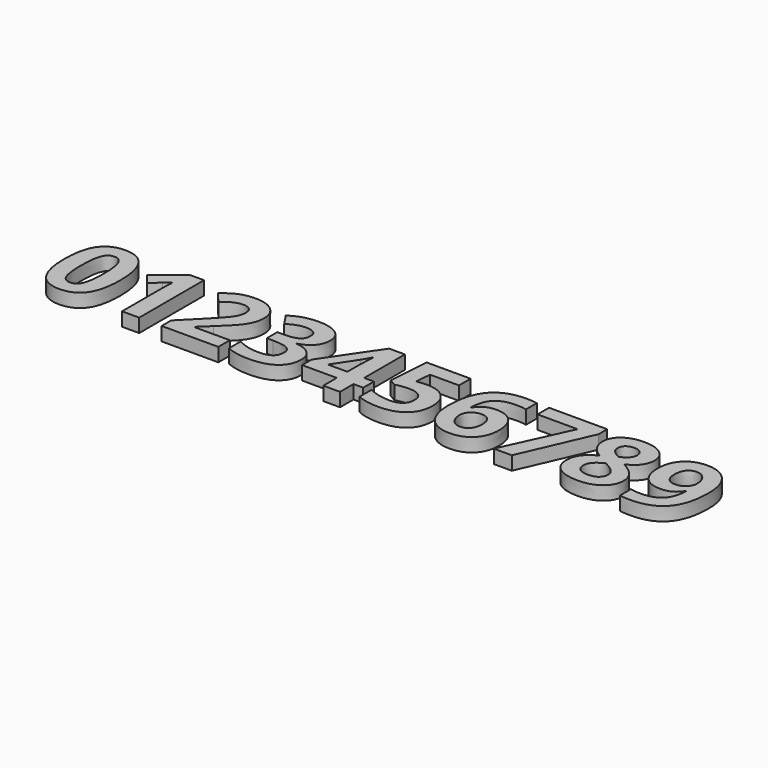
from build123d import *

# Parameters (mm, degrees)
F0_TEXT_SIZE = 16.6666666667
F1_DEPTH     = 2


# Not quite as in the source:
# - Text() gives the source's letters only with a copy of the font that has no kerning and outlines rounded to 1/6400 em; it was checked with that copy


with BuildPart() as f1:
    # F0 (on Top) → F1 (new body)
    with BuildSketch(Plane.XY):
        with Locations((0, 0)):
            Text('0123456789', F0_TEXT_SIZE, font='Open Sans', font_style=FontStyle.BOLD, text_align=(TextAlign.LEFT, TextAlign.BOTTOM))
    extrude(amount=F1_DEPTH)


solid = f1.part
